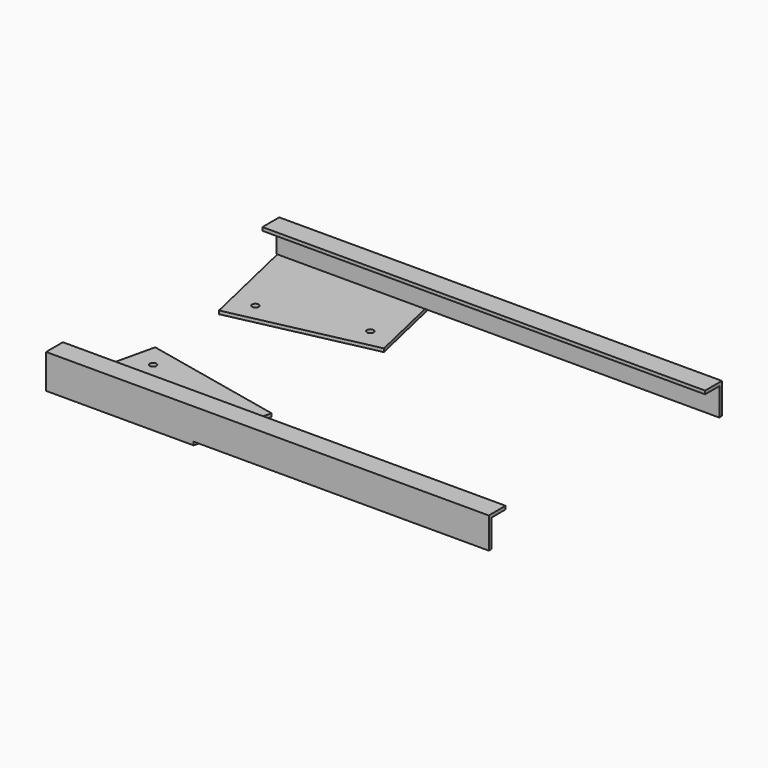
from build123d import *

# Parameters (mm, degrees)
F0_W     = 400
F0_H     = 3
F1_DEPTH = 3
F3_DEPTH = 25
F4_W     = 400
F4_H     = 3
F5_DEPTH = 28
F6_R     = 3
F7_DEPTH = 3
F8_W     = 3
F8_H     = 25
F9_DEPTH = 400.001


# Not quite as in the source:
# - a feature names something its author has since deleted; it is built from what else it names


with BuildPart() as f1:
    # F0 (on Top) → F1 (new body)
    with BuildSketch(Plane.XY):
        Polygon((-18.623991464, 31.679145366), (-218.623991464, 31.679145366), (-218.623991464, 15.679145366), (181.376008536, 15.679145366), (181.376008536, 31.679145366), align=None)
        with Locations((-18.623991464, 14.179145366)):
            Rectangle(F0_W, F0_H)
    extrude(amount=F1_DEPTH)

    # F0 (on Top) → F3 (join)
    with BuildSketch(Plane.XY):
        with Locations((-18.623991464, 14.179145366)):
            Rectangle(F0_W, F0_H)
    extrude(amount=-F3_DEPTH)

    # F4 (on face) → F5 (join)
    with BuildSketch(Plane.XY.offset(3)):
        with Locations((-18.623991464, 30.179145366)):
            Rectangle(F4_W, F4_H)
    extrude(amount=-F5_DEPTH)

    # F6 (on face) → F7 (join)
    with BuildSketch(Plane(origin=(0, 0, -25), x_dir=(1, 0, 0), z_dir=(0, 0, -1))):
        Polygon((-84.5253868028, -28.679145366), (-217.9313868906, -28.679145366), (-218.623991464, -31.679145366), (-85.2179913762, -31.679145366), align=None)
        Polygon((-69.4714175721, 36.526759169), (-196.5431985444, 63.9632764502), (-214.2380493628, -12.6815429686), (-217.9313868906, -28.679145366), (-84.5253868028, -28.679145366), (-80.9082856553, -13.0117590105), align=None)
        with Locations((-93.339475505, 22.0263727619)):
            Circle(F6_R, mode=Mode.SUBTRACT)
        with Locations((-181.0561138573, 42.1706363664)):
            Circle(F6_R, mode=Mode.SUBTRACT)
    extrude(amount=F7_DEPTH)

    # F8 (on face) → F9 (cut, through all)
    with BuildSketch(Plane.YZ.offset(181.376008536)):
        with Locations((14.179145366, -12.5)):
            Rectangle(F8_W, F8_H)
    extrude(amount=-F9_DEPTH, mode=Mode.SUBTRACT)


with BuildPart() as f10_1:
    # F10: instance of F1
    add(f1.part.mirror(Plane.XZ.offset(100)))


solid = Compound([f1.part, f10_1.part])
